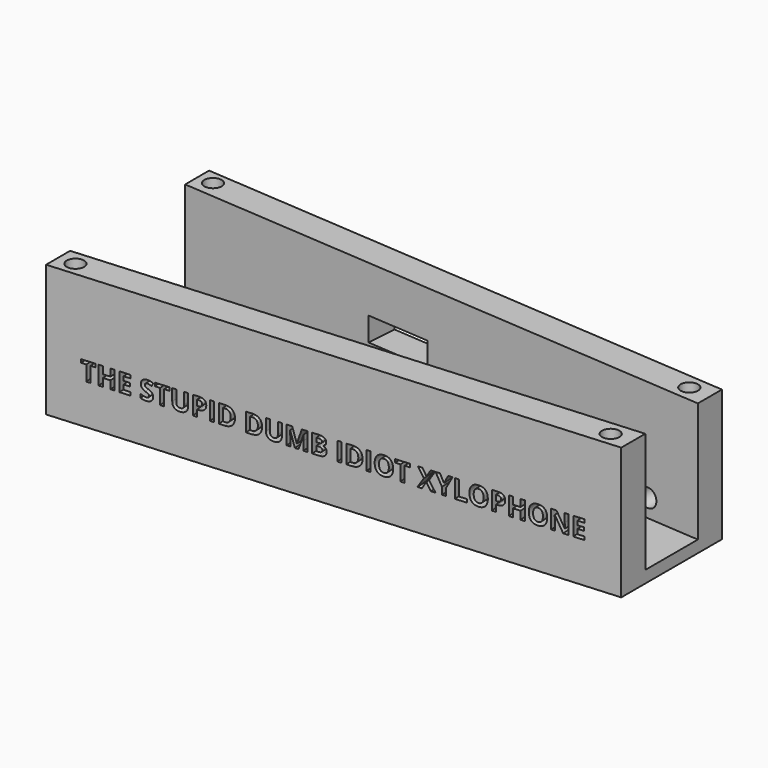
from build123d import *

# Parameters (mm, degrees)
F1_DEPTH     = 55.88
F3_DEPTH     = 50.8
F4_R         = 3.8775896532
F5_DEPTH     = 14.224
F6_W         = 26.6195088625
F6_H         = 10.0803226233
F7_DEPTH     = 15.24
F9_R         = 3.6813544887
F10_DEPTH    = 61.468
F8_TEXT_SIZE = 10.9030240533
F11_DEPTH    = 5.588


# Not quite as in the source:
# - Text() gives the source's letters only with a copy of the font that has no kerning and outlines rounded to 1/6400 em; it was checked with that copy


with BuildPart() as f1:
    # F0 (on Top) → F1 (new body)
    with BuildSketch(Plane.XY):
        Polygon((258.8796758832, 27.5891669154), (28.3300727606, 44.0991669154), (28.3300727606, -42.2608330846), (258.8796758832, -25.7508330846), align=None)
    extrude(amount=F1_DEPTH)

    # F2 (on face) → F3 (cut)
    with BuildSketch(Plane.XY.offset(55.88)):
        Polygon((258.8796758832, 14.8393902928), (28.3300727606, 31.4020204466), (28.3300727606, -29.5283106242), (258.8796758832, -13.0183106242), align=None)
    extrude(amount=-F3_DEPTH, mode=Mode.SUBTRACT)

    # F4 (on face) → F5 (cut)
    with BuildSketch(Plane(origin=(3.2864358434, 45.8925790051, 0), x_dir=(-0.9974457174, 0.0714285714, 0), z_dir=(0.0714285714, 0.9974457174, 0))):
        with Locations((-234.5948368311, 12.7342771739)):
            Circle(F4_R)
        with Locations((-207.2940915823, 13.1465229206)):
            Circle(F4_R)
        with Locations((-182.2385787964, 13.0942738615)):
            Circle(F4_R)
        with Locations((-157.5615853071, 13.7509666383)):
            Circle(F4_R)
        with Locations((-131.0250908136, 14.3216801807)):
            Circle(F4_R)
        with Locations((-103.3696234226, 14.4949248061)):
            Circle(F4_R)
        with Locations((-72.6379975677, 14.0648763627)):
            Circle(F4_R)
        with Locations((-41.0251766443, 14.1201149672)):
            Circle(F4_R)
    extrude(amount=-F5_DEPTH, mode=Mode.SUBTRACT)

    # F6 (on face) → F7 (cut)
    with BuildSketch(Plane(origin=(3.2864358434, 45.8925790051, 0), x_dir=(-0.9974457174, 0.0714285714, 0), z_dir=(0.0714285714, 0.9974457174, 0))):
        with Locations((-121.9900473952, 31.1675220728)):
            Rectangle(F6_W, F6_H)
    extrude(amount=-F7_DEPTH, mode=Mode.SUBTRACT)

    # F9 (on face) → F10 (cut)
    with BuildSketch(Plane.XY.offset(55.88)):
        with Locations((35.4733355343, -35.6573089957)):
            Circle(F9_R)
        with Locations((34.9549278617, 37.8800854087)):
            Circle(F9_R)
        with Locations((249.5386004448, 21.9892598689)):
            Circle(F9_R)
        with Locations((249.9845921993, -20.224576816)):
            Circle(F9_R)
    extrude(amount=-F10_DEPTH, mode=Mode.SUBTRACT)

    # F8 (on face) → F11 (cut)
    with BuildSketch(Plane(origin=(3.1554616857, -44.0636244285, 0), x_dir=(0.9974457174, 0.0714285714, 0), z_dir=(0.0714285714, -0.9974457174, 0))):
        with Locations((39.1019620001, 17.0179943437)):
            Text('THE STUPID DUMB IDIOT XYLOPHONE', F8_TEXT_SIZE, font='Open Sans', font_style=FontStyle.BOLD, text_align=(TextAlign.LEFT, TextAlign.BOTTOM))
    extrude(amount=-F11_DEPTH, mode=Mode.SUBTRACT)


solid = f1.part
